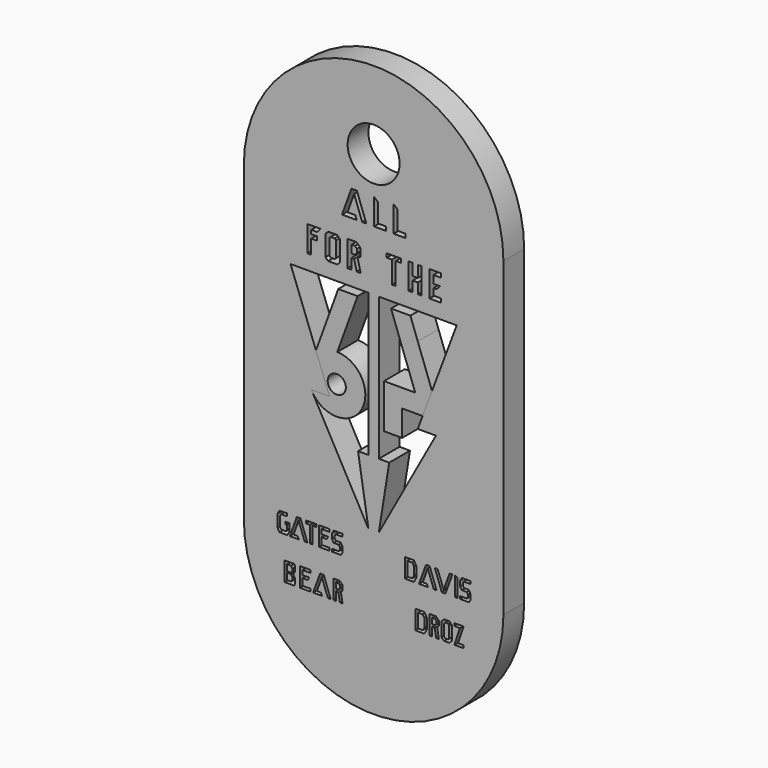
from build123d import *

# Parameters (mm, degrees)
F0_R     = 2.54
F0_W     = 25.4
F0_H     = 30.48
F1_DEPTH = 2.54
F3_DEPTH = 25.4
F4_R     = 0.889
F5_DEPTH = 2.54
F7_DEPTH = 25.4
F9_DEPTH = 25.4


# Not quite as in the source:
# - a feature names something its author has since deleted; it is built from what else it names


with BuildPart() as f1:
    # F0 (on Front) → F1 (new body)
    with BuildSketch(Plane.XZ):
        with BuildLine():
            ThreePointArc((9.902700429, -1.8280380887), (-2.797299571, 10.8719619113), (-15.497299571, -1.8280380887))
            Line((-15.497299571, -1.8280380887), (9.902700429, -1.8280380887))
        make_face()
        with Locations((-2.797299571, 3.2519619113)):
            Circle(F0_R, mode=Mode.SUBTRACT)
        with Locations((-2.797299571, -17.0680380887)):
            Rectangle(F0_W, F0_H)
        with BuildLine():
            Line((9.902700429, -32.3080380887), (-15.497299571, -32.3080380887))
            ThreePointArc((-15.497299571, -32.3080380887), (-2.797299571, -45.0080380887), (9.902700429, -32.3080380887))
        make_face()
    extrude(amount=F1_DEPTH)

    # F2 (on face) → F3 (cut)
    with BuildSketch(Plane.XZ.offset(2.54)):
        Polygon((-4.321299571, -22.8286140451), (-3.305299571, -22.8286140451), (-3.305299571, -8.8586140451), (-10.925299571, -8.8586140451), (-7.115299571, -19.0186140451), (-8.893299571, -19.0186140451), (-3.305299571, -29.1786140451), align=None)
        Polygon((5.330700429, -8.8586140451), (-2.289299571, -8.8586140451), (-2.289299571, -22.8286140451), (-1.273299571, -22.8286140451), (-2.289299571, -29.1786140451), (3.298700429, -19.0186140451), (1.520700429, -19.0186140451), align=None)
    extrude(amount=-F3_DEPTH, mode=Mode.SUBTRACT)

    # F6 (on face) → F7 (cut)
    with BuildSketch(Plane.XZ.offset(2.54)):
        Polygon((-4.9690751759, -0.4267897166), (-5.893559571, -2.9667897166), (-4.4570866765, -2.9667897166), (-4.5957593358, -2.5857897166), (-5.3494351804, -2.5857897166), (-4.7022961039, -0.8077897166), (-3.9164843681, -2.9667897166), (-3.5110326368, -2.9667897166), (-4.4355170318, -0.4267897166), align=None)
        Polygon((-2.3680326368, -0.7464866761), (-2.7490326368, -0.4267897166), (-2.7490326368, -2.9667897166), (-1.6060326368, -2.9667897166), (-1.6060326368, -2.5857897166), (-2.3680326368, -2.5857897166), align=None)
        Polygon((-0.4630326368, -0.7464866761), (-0.8440326368, -0.4267897166), (-0.8440326368, -2.9667897166), (0.2989673632, -2.9667897166), (0.2989673632, -2.5857897166), (-0.4630326368, -2.5857897166), align=None)
        Polygon((-9.2806199433, -4.8717897166), (-9.2806199433, -7.4117897166), (-8.8996199433, -7.4117897166), (-8.8996199433, -6.0147897166), (-8.3303169028, -6.0147897166), (-8.3303169028, -5.6337897166), (-8.8996199433, -5.6337897166), (-8.8996199433, -5.2527897166), (-8.3303169028, -5.2527897166), (-8.0106199433, -4.8717897166), align=None)
        Polygon((-6.3596199433, -4.8717897166), (-7.2486199433, -4.8717897166), (-7.5026199433, -5.1257897166), (-7.5026199433, -7.1577897166), (-7.2486199433, -7.4117897166), (-6.3596199433, -7.4117897166), (-6.1056199433, -7.1577897166), (-6.1056199433, -5.1257897166), align=None)
        Polygon((-6.9946199433, -7.0307897166), (-7.1216199433, -6.9037897166), (-7.1216199433, -5.3797897166), (-6.9946199433, -5.2527897166), (-6.6136199433, -5.2527897166), (-6.4866199433, -5.3797897166), (-6.4866199433, -6.9037897166), (-6.6136199433, -7.0307897166), align=None, mode=Mode.SUBTRACT)
        Polygon((-5.3436199433, -4.8717897166), (-5.3436199433, -7.4117897166), (-4.9626199433, -7.4117897166), (-4.9626199433, -6.3957897166), (-4.7086199433, -6.3957897166), (-4.4537891587, -7.4117897166), (-4.060987671, -7.4117897166), (-4.3476723037, -6.2687897166), (-4.060987671, -5.9821050838), (-4.060987671, -5.2854743493), (-4.4746723037, -4.8717897166), align=None)
        Polygon((-4.9626199433, -6.0147897166), (-4.9626199433, -5.2527897166), (-4.632487671, -5.2527897166), (-4.441987671, -5.4432897166), (-4.441987671, -5.8242897166), (-4.632487671, -6.0147897166), align=None, mode=Mode.SUBTRACT)
        Polygon((-0.123987671, -4.8717897166), (-1.520987671, -4.8717897166), (-1.520987671, -5.2527897166), (-1.012987671, -5.2527897166), (-1.012987671, -7.4117897166), (-0.631987671, -7.4117897166), (-0.631987671, -5.2527897166), (-0.123987671, -5.2527897166), align=None)
        Polygon((1.019012329, -4.8717897166), (0.638012329, -4.8717897166), (0.638012329, -7.4117897166), (1.019012329, -7.4117897166), (1.019012329, -6.3957897166), (1.527012329, -6.3957897166), (1.527012329, -7.4117897166), (1.908012329, -7.4117897166), (1.908012329, -4.8717897166), (1.527012329, -4.8717897166), (1.527012329, -6.0147897166), (1.019012329, -6.0147897166), align=None)
        Polygon((3.813012329, -4.8717897166), (2.670012329, -4.8717897166), (2.670012329, -7.4117897166), (3.813012329, -7.4117897166), (3.813012329, -7.0307897166), (3.051012329, -7.0307897166), (3.051012329, -6.3957897166), (3.3663153696, -6.3957897166), (3.686012329, -6.0147897166), (3.051012329, -6.0147897166), (3.051012329, -5.2527897166), (3.813012329, -5.2527897166), align=None)
    extrude(amount=-F7_DEPTH, mode=Mode.SUBTRACT)

    # F8 (on face) → F9 (cut)
    with BuildSketch(Plane.XZ.offset(2.54)):
        Polygon((-8.385299571, -30.4486140451), (-9.401299571, -30.4486140451), (-9.401299571, -30.7026140451), (-9.020299571, -30.7026140451), (-9.020299571, -32.3187894032), (-8.766299571, -32.3187894032), (-8.766299571, -30.7026140451), (-8.385299571, -30.7026140451), align=None)
        Polygon((-10.3106931636, -30.4486140451), (-10.9913813268, -32.3187894032), (-10.1009847647, -32.3187894032), (-10.2476317331, -32.0647894032), (-10.6286317331, -32.0647894032), (-10.1328404489, -30.7026140451), (-9.5446007252, -32.3187894032), (-9.274299571, -32.3187894032), (-9.9549877342, -30.4486140451), align=None)
        Polygon((-12.0073813268, -30.4486140451), (-12.1978813268, -30.7785697239), (-12.1978813268, -31.9888337244), (-12.0073813268, -32.3187894032), (-11.2453813268, -32.3187894032), (-11.0114873432, -31.91367314), (-11.0114873432, -31.2106140451), (-11.4432873432, -31.2106140451), (-11.4432873432, -31.4646140451), (-11.2654873432, -31.4646140451), (-11.2654873432, -31.8456140451), (-11.3670873432, -32.0215904072), (-11.8422813268, -32.0215904072), (-11.9438813268, -31.8456140451), (-11.9438813268, -30.8785904071), (-11.8422813268, -30.7026140451), (-11.2654873432, -30.7026140451), (-11.2654873432, -30.4486140451), align=None)
        Polygon((-8.131299571, -30.4486140451), (-8.131299571, -32.3187894032), (-7.115299571, -32.3187894032), (-7.115299571, -32.0647894032), (-7.877299571, -32.0647894032), (-7.877299571, -31.4043894032), (-7.3889465393, -31.4043894032), (-7.242299571, -31.1503894032), (-7.877299571, -31.1503894032), (-7.877299571, -30.7026140451), (-7.115299571, -30.7026140451), (-7.115299571, -30.4486140451), align=None)
        Polygon((-5.845299571, -30.7026140451), (-5.845299571, -30.4486140451), (-6.7027085655, -30.4486140451), (-6.861299571, -30.7233017242), (-6.861299571, -31.2313017242), (-6.7027085655, -31.5059894032), (-6.2019524488, -31.5059894032), (-6.099299571, -31.6837894032), (-6.099299571, -31.8869894032), (-6.2019524488, -32.0647894032), (-6.861299571, -32.0647894032), (-6.861299571, -32.3187894032), (-5.9919465393, -32.3187894032), (-5.845299571, -32.0647894032), (-5.845299571, -31.5567894032), (-6.021275933, -31.2519894032), (-6.5073673529, -31.2519894032), (-6.607299571, -31.0789017242), (-6.607299571, -30.8757017242), (-6.5073673529, -30.7026140451), align=None)
        Polygon((1.139700429, -30.4486140451), (0.250700429, -30.4486140451), (0.250700429, -32.3187894032), (1.139700429, -32.3187894032), (1.393700429, -31.8788484981), (1.393700429, -30.8885549502), align=None)
        Polygon((0.504700429, -32.0647894032), (0.504700429, -30.7026140451), (0.9930534607, -30.7026140451), (1.139700429, -30.9566140451), (1.139700429, -31.8107894032), (0.9930534607, -32.0647894032), align=None, mode=Mode.SUBTRACT)
        Polygon((2.3283885923, -30.4486140451), (1.647700429, -32.3187894032), (2.5380969911, -32.3187894032), (2.3914500227, -32.0647894032), (2.0104500227, -32.0647894032), (2.506241307, -30.7026140451), (3.0944810307, -32.3187894032), (3.3647821849, -32.3187894032), (2.6840940217, -30.4486140451), align=None)
        Polygon((3.4623951759, -30.4486140451), (3.1920940217, -30.4486140451), (3.8727821849, -32.3187894032), (4.2284876143, -32.3187894032), (4.9091757775, -30.4486140451), (4.6388746233, -30.4486140451), (4.0506348996, -32.0647894032), align=None)
        Polygon((-10.5764083297, -34.5754288137), (-11.5094905268, -34.5754288137), (-11.5094905268, -36.4456054137), (-10.5764083297, -36.4456054137), (-10.4934905268, -36.3019875663), (-10.4934905268, -35.7939875663), (-10.6204905268, -35.5740171137), (-10.6204905268, -35.4470171137), (-10.4934905268, -35.2270466611), (-10.4934905268, -34.7190466611), align=None)
        Polygon((-11.2554905268, -36.1916054137), (-11.2554905268, -35.5573462982), (-10.8744905268, -35.5573462982), (-10.7474905268, -35.7773167508), (-10.7474905268, -35.9716349611), (-10.8744905268, -36.1916054137), align=None, mode=Mode.SUBTRACT)
        Polygon((-11.2554905268, -35.4303547137), (-11.2554905268, -34.8294288137), (-10.8744905268, -34.8294288137), (-10.7474905268, -35.0493992663), (-10.7474905268, -35.2103842611), (-10.8744905268, -35.4303547137), align=None, mode=Mode.SUBTRACT)
        Polygon((-9.9854905268, -34.5754300556), (-9.9854905268, -36.4456054137), (-8.9694905268, -36.4456054137), (-8.9694905268, -36.1916054137), (-9.7314905268, -36.1916054137), (-9.7314905268, -35.5312054137), (-9.2431374952, -35.5312054137), (-9.0964905268, -35.2772054137), (-9.7314905268, -35.2772054137), (-9.7314905268, -34.8294300556), (-8.9694905268, -34.8294300556), (-8.9694905268, -34.5754300556), align=None)
        Polygon((-8.0348023636, -34.5754300556), (-8.7154905268, -36.4456054137), (-7.8250939647, -36.4456054137), (-7.9717409331, -36.1916054137), (-8.3527409331, -36.1916054137), (-7.8569496489, -34.8294300556), (-7.2687099252, -36.4456054137), (-6.998408771, -36.4456054137), (-7.6790969342, -34.5754300556), align=None)
        Polygon((-6.744408771, -34.5754300556), (-6.744408771, -36.4456054137), (-6.490408771, -36.4456054137), (-6.490408771, -35.6224652639), (-6.236408771, -35.6224652639), (-6.0940634713, -36.4456054137), (-5.8362935579, -36.4456054137), (-6.0006009172, -35.4954652639), (-5.8362935579, -35.3311579046), (-5.8362935579, -34.8667374149), (-6.1276009172, -34.5754300556), align=None)
        Polygon((-6.490408771, -35.3684652639), (-6.490408771, -34.8294300556), (-6.232811162, -34.8294300556), (-6.0902935579, -34.9719476597), (-6.0902935579, -35.2259476597), (-6.232811162, -35.3684652639), align=None, mode=Mode.SUBTRACT)
        Polygon((2.1696697644, -34.5754211305), (1.2806697644, -34.5754211305), (1.2806697644, -36.4455964887), (2.1696697644, -36.4455964887), (2.4236697644, -36.0056555836), (2.4236697644, -35.0153620357), align=None)
        Polygon((1.5346697644, -36.1915964887), (1.5346697644, -34.8294211305), (2.0230227961, -34.8294211305), (2.1696697644, -35.0834211305), (2.1696697644, -35.9375964887), (2.0230227961, -36.1915964887), align=None, mode=Mode.SUBTRACT)
        Polygon((2.6776697644, -34.5754211305), (2.6776697644, -36.4455964887), (2.9316697644, -36.4455964887), (2.9316697644, -35.6224563389), (3.1856697644, -35.6224563389), (3.3280150641, -36.4455964887), (3.5857849775, -36.4455964887), (3.4214776182, -35.4954563389), (3.5857849775, -35.3311489795), (3.5857849775, -34.8667284899), (3.2944776182, -34.5754211305), align=None)
        Polygon((2.9316697644, -35.3684563389), (2.9316697644, -34.8294211305), (3.1892673734, -34.8294211305), (3.3317849775, -34.9719387347), (3.3317849775, -35.2259387347), (3.1892673734, -35.3684563389), align=None, mode=Mode.SUBTRACT)
        Polygon((4.599770617, -34.5754211305), (4.091770617, -34.5754211305), (3.8397849775, -34.8314251088), (3.8397849775, -36.1915964887), (4.0937849775, -36.4455964887), (4.6017849775, -36.4455964887), (4.8557849775, -36.1915964887), (4.8557849775, -34.8273962217), align=None)
        Polygon((4.0937849775, -36.0863862438), (4.0937849775, -34.9354603001), (4.1981597147, -34.8294211305), (4.4957415075, -34.8294211305), (4.6017849775, -34.9337914985), (4.6017849775, -36.0863862438), (4.4965747327, -36.1915964887), (4.1989952224, -36.1915964887), align=None, mode=Mode.SUBTRACT)
        Polygon((5.9987849775, -34.5754211305), (5.1097849775, -34.5754211305), (5.1097849775, -34.8294211305), (5.6467440061, -34.8294211305), (5.1097849775, -36.4455964887), (5.9987849775, -36.4455964887), (5.9987849775, -36.1915964887), (5.4618259489, -36.1915964887), align=None)
        Polygon((5.4171757775, -30.5952610135), (5.1631757775, -30.4486140451), (5.1631757775, -32.3187894032), (5.4171757775, -32.3187894032), align=None)
        Polygon((6.6871757775, -30.7026140451), (6.6871757775, -30.4486140451), (5.829766783, -30.4486140451), (5.6711757775, -30.7233017242), (5.6711757775, -31.2313017242), (5.829766783, -31.5059894032), (6.3305228997, -31.5059894032), (6.4331757775, -31.6837894032), (6.4331757775, -31.8869894032), (6.3305228997, -32.0647894032), (5.6711757775, -32.0647894032), (5.6711757775, -32.3187894032), (6.5405288092, -32.3187894032), (6.6871757775, -32.0647894032), (6.6871757775, -31.5567894032), (6.5111994155, -31.2519894032), (6.0251079956, -31.2519894032), (5.9251757775, -31.0789017242), (5.9251757775, -30.8757017242), (6.0251079956, -30.7026140451), align=None)
    extrude(amount=-F9_DEPTH, mode=Mode.SUBTRACT)


with BuildPart() as f5:
    # F4 (on face) → F5 (new body)
    with BuildSketch(Plane.XZ.offset(2.54)):
        with BuildLine():
            ThreePointArc((-8.3448988742, -15.7396825699), (-7.42721995, -15.1490776832), (-6.353299571, -14.9550576855))
            Line((-6.353299571, -14.9550576855), (-4.3654966497, -9.4936140451))
            Line((-4.3654966497, -9.4936140451), (-6.2576047292, -9.4936140451))
            Line((-6.2576047292, -9.4936140451), (-8.439332082, -15.4878606823))
            Line((-8.439332082, -15.4878606823), (-8.3448988742, -15.7396825699))
        make_face()
        with BuildLine():
            ThreePointArc((-8.8512350228, -19.0950950418), (-5.7079933247, -20.4547699347), (-3.6090877793, -17.7486140451))
            ThreePointArc((-3.6090877793, -17.7486140451), (-4.4099063709, -15.790639614), (-6.353299571, -14.9550576855))
            ThreePointArc((-6.353299571, -14.9550576855), (-7.42721995, -15.1490776832), (-8.3448988742, -15.7396825699))
            Line((-8.3448988742, -15.7396825699), (-7.115299571, -19.0186140451))
            Line((-7.115299571, -19.0186140451), (-8.891769358, -19.0186140451))
            ThreePointArc((-8.891769358, -19.0186140451), (-8.8717983821, -19.0570115228), (-8.8512350228, -19.0950950418))
        make_face()
        with Locations((-6.4030877793, -17.7486140451)):
            Circle(F4_R, mode=Mode.SUBTRACT)
    extrude(amount=-F5_DEPTH)


with BuildPart() as f5b:
    # F4 (on face) → F5, piece 2 (new body)
    with BuildSketch(Plane.XZ.offset(2.54)):
        Polygon((-1.781299571, -15.9706140451), (-1.781299571, -20.2886140451), (-0.003299571, -20.2886140451), (-0.003299571, -17.7486140451), (1.996950429, -17.7486140451), (2.915331466, -15.2995979466), (1.520700429, -11.4678806642), (0.8021261452, -9.4936140451), (-1.0899819343, -9.4936140451), (0.1311473049, -12.8486390559), (1.267453273, -15.9706140451), align=None)
    extrude(amount=-F5_DEPTH)


solid = Compound([f1.part, f5.part, f5b.part])
